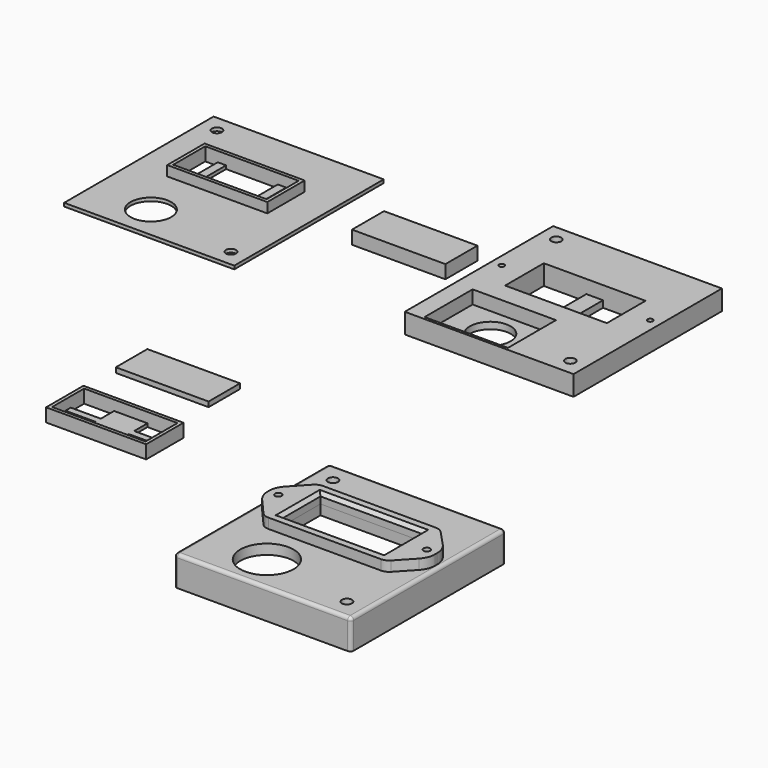
from build123d import *

# Parameters (mm, degrees)
F0_W      = 51
F0_H      = 56
F0_R      = 1.5
F0_R_2    = 6.1
F0_W_2    = 5
F0_H_2    = 14.5
F1_DEPTH  = 1
F0_W_3    = 2.5
F0_H_3    = 12
F3_W      = 28
F3_H      = 1
F4_DEPTH  = 3
F5_W      = 28
F5_H      = 12
F6_DEPTH  = 4
F7_T      = -1
F8_W      = 2
F8_H      = 10
F9_DEPTH  = 3
F2_W      = 30
F2_H      = 14
F11_DEPTH = 4
F2_W_2    = 51
F2_H_2    = 56
F2_R      = 8
F2_R_2    = 1.5
F2_R_3    = 0.8
F2_W_3    = 30.5
F2_H_3    = 14.5
F12_DEPTH = 3
F2_W_4    = 9
F2_H_4    = 2
F2_W_5    = 10
F2_H_5    = 5
F13_DEPTH = 1
F5_W_2    = 27.8
F5_H_2    = 11.8
F14_DEPTH = 1.5
F2_H_6    = 1
F15_DEPTH = 9
F16_W     = 36.5
F16_H     = 20.5
F16_W_2   = 30.5
F16_H_2   = 14.5
F16_R     = 1
F17_DEPTH = 3
F18_R     = 6
F19_R     = 3
F20_R     = 1
F21_SIZE  = 1
F24_DEPTH = 1
F25_D     = 1.4
F25_DEPTH = 1.001
F27_D     = 1.4
F22_W     = 51
F22_H     = 56
F22_W_2   = 25
F22_H_2   = 18
F22_R     = 1.5
F28_DEPTH = 5
F29_W     = 0.2
F29_H     = 55.6
F30_DEPTH = 25
F31_D     = 1.6
F31_DEPTH = 5.001
F32_D     = 1.6


# Not quite as in the source:
# - a feature names something its author has since deleted; it is built from what else it names


with BuildPart() as f1:
    # F0 (on Top) → F1 (new body)
    with BuildSketch(Plane.XY):
        Rectangle(F0_W, F0_H)
        with Locations((20.5, -23)):
            Circle(F0_R, mode=Mode.SUBTRACT)
        with Locations((-7.5, -18)):
            Circle(F0_R_2, mode=Mode.SUBTRACT)
        Polygon((-15.25, -2.75), (-15.25, 11.75), (-2.5, 11.75), (2.5, 11.75), (15.25, 11.75), (15.25, -2.75), (2.5, -2.75), (-2.5, -2.75), align=None, mode=Mode.SUBTRACT)
        with Locations((-20.5, 23)):
            Circle(F0_R, mode=Mode.SUBTRACT)
        with Locations((0, 4.5)):
            Rectangle(F0_W_2, F0_H_2)
    extrude(amount=F1_DEPTH)

    # F24 (add): a face of the model
    f24_faces = [f1.faces().sort_by_distance(p)[0] for p in [
        (0.3722548806, 0.1869472989, 1),
    ]]
    extrude(f24_faces, amount=F24_DEPTH)

    # F25 (through all, one way)
    with BuildSketch(Plane.XY.offset(1)):
        with Locations((-22.25, 4.75), (22.25, 4.75)):
            Circle(F25_D / 2)
    extrude(amount=-F25_DEPTH, mode=Mode.SUBTRACT)

    # F27 (through all)
    with Locations(Plane(origin=(0, 0, 1), x_dir=(1, 0, 0), z_dir=(0, 0, -1))):
        with Locations((-22.25, -4.75), (22.25, -4.75)):
            Hole(F27_D / 2)

    # F22 (on face) → F28 (join)
    with BuildSketch(Plane.XY.offset(1)):
        Rectangle(F22_W, F22_H)
        with Locations((-7.5, -18)):
            Rectangle(F22_W_2, F22_H_2, mode=Mode.SUBTRACT)
        with Locations((20.5, -23)):
            Circle(F22_R, mode=Mode.SUBTRACT)
        with Locations((-20.5, 23)):
            Circle(F22_R, mode=Mode.SUBTRACT)
        Polygon((-15.25, -2.75), (-15.25, 11.75), (-2.5, 11.75), (2.5, 11.75), (15.25, 11.75), (15.25, -2.75), (2.5, -2.75), (-2.5, -2.75), align=None, mode=Mode.SUBTRACT)
    extrude(amount=F28_DEPTH)

    # F29 (on face) → F30 (cut)
    with BuildSketch(Plane(origin=(0, 0, 0), x_dir=(1, 0, 0), z_dir=(0, 0, -1))):
        Polygon((25.5, 28), (-25.5, 28), (-25.5, 27.8), (-25.3, 27.8), (25.3, 27.8), (25.5, 27.8), align=None)
        with Locations((-25.4, 0)):
            Rectangle(F29_W, F29_H)
        with Locations((25.4, 0)):
            Rectangle(F29_W, F29_H)
        Polygon((-25.3, -27.8), (-25.5, -27.8), (-25.5, -28), (25.5, -28), (25.5, -27.8), (25.3, -27.8), align=None)
    extrude(amount=-F30_DEPTH, mode=Mode.SUBTRACT)

    # F31 (through all, one way)
    with BuildSketch(Plane(origin=(0, 0, 1), x_dir=(1, 0, 0), z_dir=(0, 0, -1))):
        with Locations((-22.25, -4.75), (22.25, -4.75)):
            Circle(F31_D / 2)
    extrude(amount=-F31_DEPTH, mode=Mode.SUBTRACT)

    # F32 (through all)
    with Locations(Plane.XY.offset(1)):
        with Locations((22.25, 4.75), (-22.25, 4.75)):
            Hole(F32_D / 2)


with BuildPart() as f1b:
    # F0 (on Top) → F1, piece 2 (new body)
    with BuildSketch(Plane.XY):
        with Locations((-102.5748546124, 1.0383715183)):
            Rectangle(F0_W, F0_H)
        with Locations((-110.0748546124, -16.9616284817)):
            Circle(F0_R_2, mode=Mode.SUBTRACT)
        with Locations((-82.0748546124, -21.9616284817)):
            Circle(F0_R, mode=Mode.SUBTRACT)
        Polygon((-116.5748546124, -0.4616284817), (-116.5748546124, 11.5383715183), (-112.8248546124, 11.5383715183), (-110.3248546124, 11.5383715183), (-94.8248546124, 11.5383715183), (-92.3248546124, 11.5383715183), (-88.5748546124, 11.5383715183), (-88.5748546124, -0.4616284817), (-92.3248546124, -0.4616284817), (-94.8248546124, -0.4616284817), (-110.3248546124, -0.4616284817), (-112.8248546124, -0.4616284817), align=None, mode=Mode.SUBTRACT)
        with Locations((-123.0748546124, 24.0383715183)):
            Circle(F0_R, mode=Mode.SUBTRACT)
        with Locations((-111.5748546124, 5.5383715183)):
            Rectangle(F0_W_3, F0_H_3)
        with Locations((-93.5748546124, 5.5383715183)):
            Rectangle(F0_W_3, F0_H_3)
    extrude(amount=F1_DEPTH)

    # F3 (on face) → F4 (join)
    with BuildSketch(Plane.XY.offset(1)):
        with Locations((-102.5748546124, 12.0383715183)):
            Rectangle(F3_W, F3_H)
        Polygon((-116.5748546124, -0.4616284817), (-116.5748546124, 11.5383715183), (-116.5748546124, 12.5383715183), (-117.5748546124, 12.5383715183), (-117.5748546124, -1.4616284817), (-116.5748546124, -1.4616284817), align=None)
        Polygon((-88.5748546124, 12.5383715183), (-88.5748546124, 11.5383715183), (-88.5748546124, -0.4616284817), (-88.5748546124, -1.4616284817), (-87.5748546124, -1.4616284817), (-87.5748546124, 12.5383715183), align=None)
        with Locations((-102.5748546124, -0.9616284817)):
            Rectangle(F3_W, F3_H)
    extrude(amount=F4_DEPTH)


with BuildPart() as f6:
    # F5 (on Top) → F6 (new body)
    with BuildSketch(Plane.XY):
        with Locations((-49.3556470275, 6)):
            Rectangle(F5_W, F5_H)
    extrude(amount=F6_DEPTH)

    # F7
    f7_openings = [f6.faces().sort_by_distance(p)[0] for p in [
        (-49.355647, 6, 0),
    ]]
    offset(amount=F7_T, openings=f7_openings)

    # F8 (on face) → F9 (join)
    with BuildSketch(Plane(origin=(0, 0, 3), x_dir=(1, 0, 0), z_dir=(0, 0, -1))):
        with Locations((-49.3556470275, -6)):
            Rectangle(F8_W, F8_H)
    extrude(amount=F9_DEPTH)


with BuildPart() as f11:
    # F2 (on Top) → F11 (new body)
    with BuildSketch(Plane.XY):
        with Locations((-48.0005137329, -108.0776734079)):
            Rectangle(F2_W, F2_H)
        Polygon((-62.0005137329, -107.0776734079), (-62.0005137329, -102.0776734079), (-53.0005137329, -102.0776734079), (-43.0005137329, -102.0776734079), (-34.0005137329, -102.0776734079), (-34.0005137329, -107.0776734079), (-34.0005137329, -109.0776734079), (-34.0005137329, -114.0776734079), (-43.0005137329, -114.0776734079), (-53.0005137329, -114.0776734079), (-62.0005137329, -114.0776734079), (-62.0005137329, -109.0776734079), align=None, mode=Mode.SUBTRACT)
    extrude(amount=F11_DEPTH)

    # F2 (on Top) → F13 (join)
    with BuildSketch(Plane.XY):
        with Locations((-57.5005137329, -108.0776734079)):
            Rectangle(F2_W_4, F2_H_4)
        with Locations((-48.0005137329, -108.0776734079)):
            Rectangle(F2_W_5, F2_H_4)
        with Locations((-38.5005137329, -108.0776734079)):
            Rectangle(F2_W_4, F2_H_4)
        with Locations((-48.0005137329, -104.5776734079)):
            Rectangle(F2_W_5, F2_H_5)
        with Locations((-48.0005137329, -111.5776734079)):
            Rectangle(F2_W_5, F2_H_5)
    extrude(amount=F13_DEPTH)


with BuildPart() as f12:
    # F2 (on Top) → F12 (new body)
    with BuildSketch(Plane.XY):
        with Locations((28.2103444552, -118.9687541723)):
            Rectangle(F2_W_2, F2_H_2)
        with Locations((20.7103444552, -136.9687541723)):
            Circle(F2_R, mode=Mode.SUBTRACT)
        with Locations((48.7103444552, -141.9687541723)):
            Circle(F2_R_2, mode=Mode.SUBTRACT)
        with Locations((5.9603444552, -114.2187541723)):
            Circle(F2_R_3, mode=Mode.SUBTRACT)
        with Locations((28.2103444552, -114.4687541723)):
            Rectangle(F2_W_3, F2_H_3, mode=Mode.SUBTRACT)
        with Locations((50.4603444552, -114.2187541723)):
            Circle(F2_R_3, mode=Mode.SUBTRACT)
        with Locations((7.7103444552, -95.9687541723)):
            Circle(F2_R_2, mode=Mode.SUBTRACT)
    extrude(amount=-F12_DEPTH)

    # F2 (on Top) → F15 (join)
    with BuildSketch(Plane.XY):
        Polygon((2.7103444552, -146.9687541723), (2.7103444552, -90.9687541723), (2.7103444552, -89.9687541723), (1.7103444552, -89.9687541723), (1.7103444552, -147.9687541723), (2.7103444552, -147.9687541723), align=None)
        with Locations((28.2103444552, -90.4687541723)):
            Rectangle(F2_W_2, F2_H_6)
        with Locations((28.2103444552, -147.4687541723)):
            Rectangle(F2_W_2, F2_H_6)
        Polygon((53.7103444552, -89.9687541723), (53.7103444552, -90.9687541723), (53.7103444552, -146.9687541723), (53.7103444552, -147.9687541723), (54.7103444552, -147.9687541723), (54.7103444552, -89.9687541723), align=None)
    extrude(amount=-F15_DEPTH)

    # F20
    f20_edges = [f12.edges().sort_by_distance(p)[0] for p in [
        (1.710344, -118.968754, 0),
        (28.210344, -89.968754, 0),
        (28.210344, -147.968754, 0),
        (54.710344, -118.968754, 0),
        (54.710344, -147.968754, -4.5),
        (1.710344, -147.968754, -4.5),
        (1.710344, -89.968754, -4.5),
        (54.710344, -89.968754, -4.5),
    ]]
    fillet(f20_edges, radius=F20_R)


with BuildPart() as f14:
    # F5 (on Top) → F14 (new body)
    with BuildSketch(Plane.XY):
        with Locations((-52.0366017878, -79.3675661445)):
            Rectangle(F5_W_2, F5_H_2)
    extrude(amount=F14_DEPTH)


with BuildPart() as f17:
    # F16 (on face) → F17 (new body)
    with BuildSketch(Plane.XY):
        with Locations((28.2103444552, -114.4687541723)):
            Rectangle(F16_W, F16_H)
        with Locations((28.2103444552, -114.4687541723)):
            Rectangle(F16_W_2, F16_H_2, mode=Mode.SUBTRACT)
        Polygon((9.9603444552, -124.7187541723), (9.9603444552, -104.2187541723), (2.9603444552, -111.7187541723), (2.9603444552, -116.7187541723), align=None)
        with Locations((5.9603444552, -114.2187541723)):
            Circle(F16_R, mode=Mode.SUBTRACT)
        Polygon((53.4603444552, -111.7187541723), (46.4603444552, -104.2187541723), (46.4603444552, -124.7187541723), (53.4603444552, -117.2187541723), align=None)
        with Locations((50.4603444552, -114.2187541723)):
            Circle(F16_R, mode=Mode.SUBTRACT)
    extrude(amount=F17_DEPTH)

    # F18
    f18_edges = [f17.edges().sort_by_distance(p)[0] for p in [
        (2.960344, -111.718754, 1.5),
        (2.960344, -116.718754, 1.5),
        (53.460344, -117.218754, 1.5),
        (53.460344, -111.718754, 1.5),
    ]]
    fillet(f18_edges, radius=F18_R)

    # F19
    f19_edges = [f17.edges().sort_by_distance(p)[0] for p in [
        (9.960344, -104.218754, 1.5),
        (9.960344, -124.718754, 1.5),
        (46.460344, -124.718754, 1.5),
        (46.460344, -104.218754, 1.5),
    ]]
    fillet(f19_edges, radius=F19_R)

    # F21
    f21_edges = [f17.edges().sort_by_distance(p)[0] for p in [
        (12.960344, -114.468754, 3),
        (28.210344, -107.218754, 3),
        (43.460344, -114.468754, 3),
        (28.210344, -121.718754, 3),
    ]]
    chamfer(f21_edges, length=F21_SIZE)


solid = Compound([f1.part, f1b.part, f6.part, f11.part, f12.part, f14.part, f17.part])
